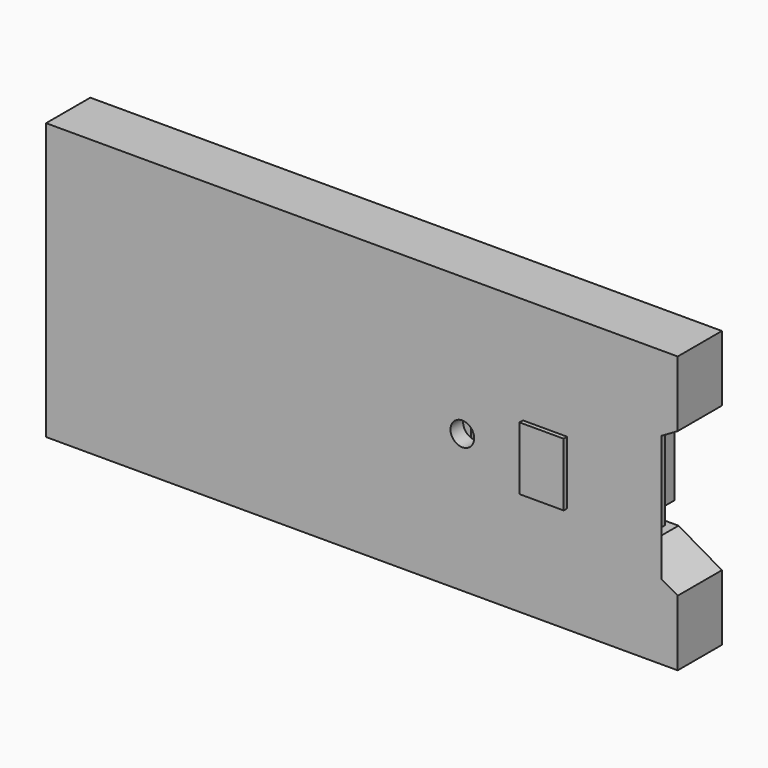
from build123d import *

# Parameters (mm, degrees)
F0_W      = 36
F0_H      = 12.4
F0_R      = 1.1
F0_W_2    = 4.4
F0_H_2    = 7.8
F0_W_3    = 12.5
F0_H_3    = 11
F1_DEPTH  = 1.55
F2_DEPTH  = 2
F0_W_4    = 1.15
F3_DEPTH  = 2.9
F0_W_5    = 3.5
F4_DEPTH  = 1.5
F5_DEPTH  = 1.3
F6_R      = 1
F7_DEPTH  = 3
F8_W      = 5.6
F8_H      = 8
F10_DEPTH = 4.5
F9_W      = 1.5
F9_H      = 10
F11_DEPTH = 1.4
F9_W_2    = 6.5
F12_DEPTH = 2.5
F13_W     = 80
F13_H     = 35
F14_DEPTH = 7
F15_W     = 7
F15_H     = 10
F16_DEPTH = 2
F15_W_2   = 4
F15_H_2   = 1.5
F17_DEPTH = 5.45
F18_DEPTH = 3.95
F19_R     = 1.5
F20_DEPTH = 2
F21_W     = 5
F21_H     = 12
F22_DEPTH = 5.5
F22_TAPER = -30


with BuildPart() as f1:
    # F0 (on Front) → F1 (new body)
    with BuildSketch(Plane.XZ):
        Polygon((-30.5, -8.95), (30.5, -8.95), (30.5, -5.5), (18, -5.5), (18, 5.5), (30.5, 5.5), (30.5, 8.95), (-30.5, 8.95), (-30.5, 3.9), (-26.1, 3.9), (-26.1, -3.9), (-30.5, -3.9), align=None)
        with Locations((-7.5, 0)):
            Rectangle(F0_W, F0_H, mode=Mode.SUBTRACT)
        with Locations((12.72, 0)):
            Circle(F0_R, mode=Mode.SUBTRACT)
        with Locations((-28.3, 0)):
            Rectangle(F0_W_2, F0_H_2)
        with Locations((24.25, 0)):
            Rectangle(F0_W_3, F0_H_3)
        with Locations((12.72, 0)):
            Circle(F0_R)
        with Locations((-7.5, 0)):
            Rectangle(F0_W, F0_H)
    extrude(amount=-F1_DEPTH)

    # F0 (on Front) → F2 (join)
    with BuildSketch(Plane.XZ):
        with Locations((12.72, 0)):
            Circle(F0_R)
    extrude(amount=F2_DEPTH)

    # F0 (on Front) → F3 (join)
    with BuildSketch(Plane.XZ):
        with Locations((-28.3, 0)):
            Rectangle(F0_W_2, F0_H_2)
        with Locations((-31.075, 0)):
            Rectangle(F0_W_4, F0_H_2)
    extrude(amount=F3_DEPTH)

    # F0 (on Front) → F4 (join)
    with BuildSketch(Plane.XZ):
        with Locations((32.25, 0)):
            Rectangle(F0_W_5, F0_H_3)
        with Locations((24.25, 0)):
            Rectangle(F0_W_3, F0_H_3)
    extrude(amount=F4_DEPTH)

    # F0 (on Front) → F5 (join)
    with BuildSketch(Plane.XZ):
        with Locations((-7.5, 0)):
            Rectangle(F0_W, F0_H)
    extrude(amount=F5_DEPTH)

    # F6 (on face) → F7 (join)
    with BuildSketch(Plane(origin=(0, 1.55, 0), x_dir=(-1, 0, 0), z_dir=(0, 1, 0))):
        with Locations((29.21, -7.62)):
            Circle(F6_R)
        with Locations((29.21, 7.62)):
            Circle(F6_R)
        with Locations((26.67, -7.62)):
            Circle(F6_R)
        with Locations((26.67, 7.62)):
            Circle(F6_R)
        with Locations((24.13, -7.62)):
            Circle(F6_R)
        with Locations((24.13, 7.62)):
            Circle(F6_R)
        with Locations((21.59, -7.62)):
            Circle(F6_R)
        with Locations((21.59, 7.62)):
            Circle(F6_R)
        with Locations((19.05, -7.62)):
            Circle(F6_R)
        with Locations((19.05, 7.62)):
            Circle(F6_R)
        with Locations((16.51, -7.62)):
            Circle(F6_R)
        with Locations((16.51, 7.62)):
            Circle(F6_R)
        with Locations((13.97, -7.62)):
            Circle(F6_R)
        with Locations((13.97, 7.62)):
            Circle(F6_R)
        with Locations((11.43, -7.62)):
            Circle(F6_R)
        with Locations((11.43, 7.62)):
            Circle(F6_R)
        with Locations((8.89, -7.62)):
            Circle(F6_R)
        with Locations((8.89, 7.62)):
            Circle(F6_R)
        with Locations((6.35, -7.62)):
            Circle(F6_R)
        with Locations((6.35, 7.62)):
            Circle(F6_R)
        with Locations((3.81, -7.62)):
            Circle(F6_R)
        with Locations((3.81, 7.62)):
            Circle(F6_R)
        with Locations((1.27, -7.62)):
            Circle(F6_R)
        with Locations((1.27, 7.62)):
            Circle(F6_R)
        with Locations((-1.27, -7.62)):
            Circle(F6_R)
        with Locations((-1.27, 7.62)):
            Circle(F6_R)
        with Locations((-3.81, -7.62)):
            Circle(F6_R)
        with Locations((-3.81, 7.62)):
            Circle(F6_R)
        with Locations((-6.35, -7.62)):
            Circle(F6_R)
        with Locations((-6.35, 7.62)):
            Circle(F6_R)
        with Locations((-8.89, -7.62)):
            Circle(F6_R)
        with Locations((-8.89, 7.62)):
            Circle(F6_R)
        with Locations((-11.43, -7.62)):
            Circle(F6_R)
        with Locations((-11.43, 7.62)):
            Circle(F6_R)
        with Locations((-13.97, -7.62)):
            Circle(F6_R)
        with Locations((-13.97, 7.62)):
            Circle(F6_R)
        with Locations((-16.51, -7.62)):
            Circle(F6_R)
        with Locations((-16.51, 7.62)):
            Circle(F6_R)
        with Locations((-19.05, -7.62)):
            Circle(F6_R)
        with Locations((-19.05, 7.62)):
            Circle(F6_R)
        with Locations((-21.59, -7.62)):
            Circle(F6_R)
        with Locations((-21.59, 7.62)):
            Circle(F6_R)
        with Locations((-24.13, -7.62)):
            Circle(F6_R)
        with Locations((-24.13, 7.62)):
            Circle(F6_R)
        with Locations((-26.67, -7.62)):
            Circle(F6_R)
        with Locations((-26.67, 7.62)):
            Circle(F6_R)
        with Locations((-29.21, -7.62)):
            Circle(F6_R)
        with Locations((-29.21, 7.62)):
            Circle(F6_R)
    extrude(amount=F7_DEPTH)


with BuildPart() as f10:
    # F8 (on face) → F10 (new body)
    with BuildSketch(Plane.XZ.offset(1.5)):
        with Locations((23.2, 0)):
            Rectangle(F8_W, F8_H)
    extrude(amount=F10_DEPTH)


with BuildPart() as f11:
    # F9 (on face) → F11 (new body)
    with BuildSketch(Plane(origin=(0, 1.55, 0), x_dir=(-1, 0, 0), z_dir=(0, 1, 0))):
        with Locations((-31.25, 0)):
            Rectangle(F9_W, F9_H)
    extrude(amount=-F11_DEPTH)

    # F9 (on face) → F12 (join)
    with BuildSketch(Plane(origin=(0, 1.55, 0), x_dir=(-1, 0, 0), z_dir=(0, 1, 0))):
        with Locations((-31.25, 0)):
            Rectangle(F9_W, F9_H)
        with Locations((-27.25, 0)):
            Rectangle(F9_W_2, F9_H)
    extrude(amount=F12_DEPTH)


with BuildPart() as f14:
    # F13 (on face) → F14 (new body)
    with BuildSketch(Plane(origin=(0, 1.55, 0), x_dir=(-1, 0, 0), z_dir=(0, 1, 0))):
        Rectangle(F13_W, F13_H)
        Polygon((-34.5, 6), (-31, 6), (-31, 9.45), (31, 9.45), (31, 4.4), (32.15, 4.4), (32.15, -4.4), (31, -4.4), (31, -9.45), (-31, -9.45), (-31, -6), (-34.5, -6), align=None, mode=Mode.SUBTRACT)
    extrude(amount=-F14_DEPTH)

    # F15 (on face) → F16 (join)
    with BuildSketch(Plane.XZ.offset(5.45)):
        Polygon((-31, 9.45), (-31, 6.1), (-27, 6.1), (-27, 4.6), (-31, 4.6), (-31, 4.4), (-32.15, 4.4), (-32.15, -4.4), (-31, -4.4), (-31, -4.6), (-27, -4.6), (-27, -6.1), (-31, -6.1), (-31, -9.45), (31, -9.45), (31, -6), (34.5, -6), (34.5, 6), (31, 6), (31, 9.45), align=None)
        with Locations((26.5, 0)):
            Rectangle(F15_W, F15_H, mode=Mode.SUBTRACT)
    extrude(amount=-F16_DEPTH)

    # F15 (on face) → F17 (join, through all)
    with BuildSketch(Plane.XZ.offset(5.45)):
        with Locations((-29, 5.35)):
            Rectangle(F15_W_2, F15_H_2)
        with Locations((-29, -5.35)):
            Rectangle(F15_W_2, F15_H_2)
    extrude(amount=-F17_DEPTH)

    # F15 (on face) → F18 (join, through all)
    with BuildSketch(Plane.XZ.offset(5.45)):
        with Locations((26.5, 0)):
            Rectangle(F15_W, F15_H)
    extrude(amount=-F18_DEPTH)

    # F19 (on face) → F20 (cut, through all)
    with BuildSketch(Plane.XZ.offset(5.45)):
        with Locations((12.72, 0)):
            Circle(F19_R)
    extrude(amount=-F20_DEPTH, mode=Mode.SUBTRACT)

    # F21 (on face) → F22 (cut, through all)
    with BuildSketch(Plane(origin=(34.5, 0, 0), x_dir=(0, -1, 0), z_dir=(-1, 0, 0))):
        with Locations((0.95, 0)):
            Rectangle(F21_W, F21_H)
    extrude(amount=-F22_DEPTH, taper=F22_TAPER, mode=Mode.SUBTRACT)


solid = Compound([f1.part, f10.part, f11.part, f14.part])
